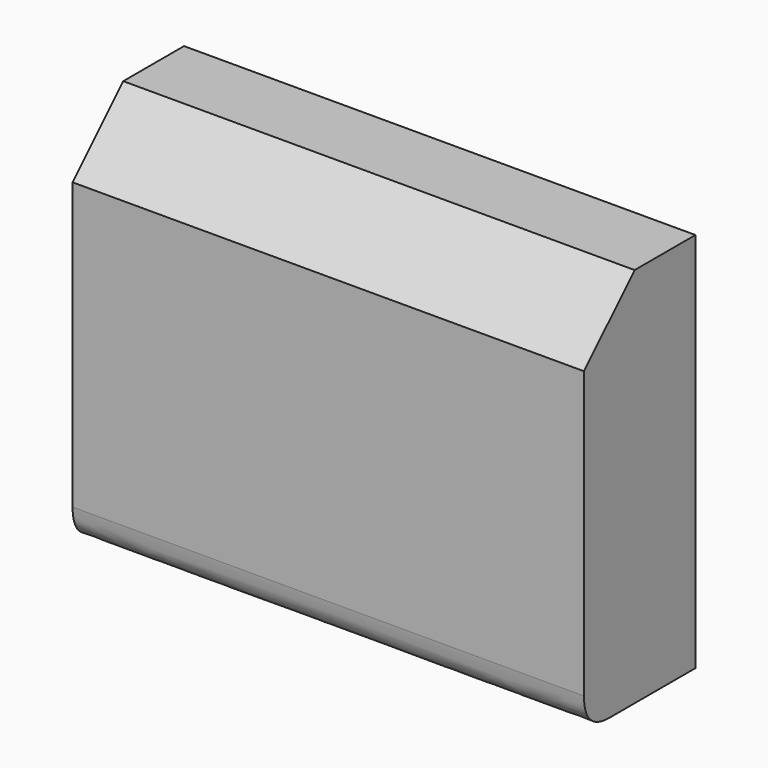
from build123d import *

# Parameters (mm, degrees)
F0_W        = 80.775000155
F0_H        = 60.2360032499
F1_DEPTH    = 22
F2_T1_DEPTH = 106.175000155
F3_SIZE     = 10


# Not quite as in the source:
# - a fillet or chamfer that OpenCascade refuses, or shapes differently, is made with other operations: its cross-section is extruded or revolved along the edge and cut away or added


with BuildPart() as f1:
    # F0 (on Front) → F1 (new body)
    with BuildSketch(Plane.XZ):
        with Locations((0.7447451353, -30.1180016249)):
            Rectangle(F0_W, F0_H)
    extrude(amount=F1_DEPTH)

    # F2: fillet of radius 5.08 on 1 edges, made by hand

    # F2_s2 → F2_t1 (cut)
    with BuildSketch(Plane.YZ.offset(-52.3427549422)):
        with BuildLine():
            add(Edge.make_bspline(
                [(-16.92, -60.2360032499), (-22, -60.2360032499), (-22, -55.1560032499)],
                knots=[0, 0, 0, 1, 1, 1], degree=2, weights=[1, 1, 1]))
            Line((-22, -55.1560032499), (-22, -60.2360032499))
            Line((-22, -60.2360032499), (-16.92, -60.2360032499))
        make_face()
    extrude(amount=F2_T1_DEPTH, mode=Mode.SUBTRACT)

    # F3
    f3_edges = [f1.edges().sort_by_distance(p)[0] for p in [
        (0.744745, -22, 0),
    ]]
    chamfer(f3_edges, length=F3_SIZE)


solid = f1.part
